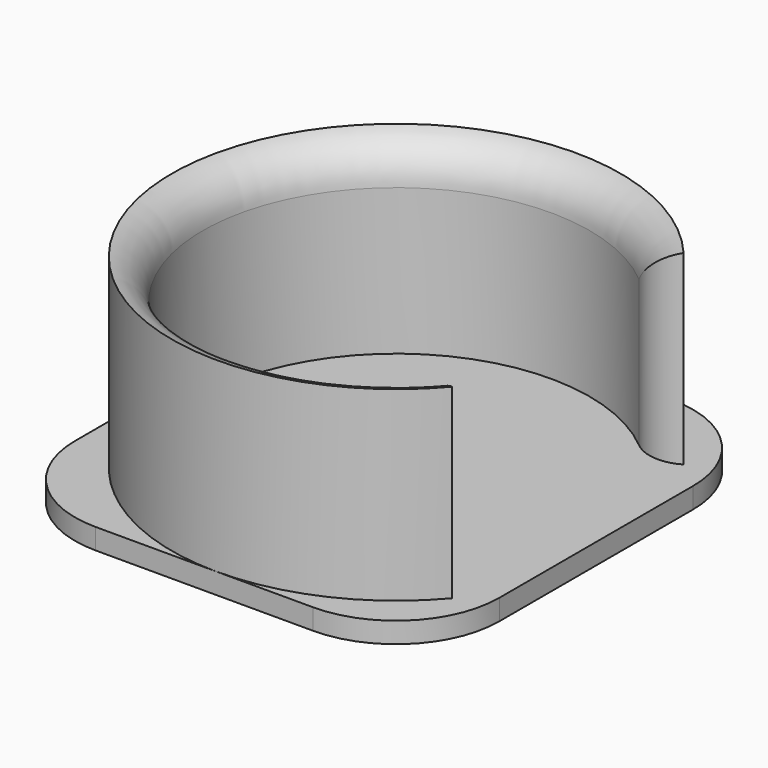
from build123d import *

# Parameters (mm, degrees)
F2_DEPTH    = 10
F3_W        = 20.5154874287
F3_H        = 21.7
F4_DEPTH    = 1
F5_R        = 5
F7_T1_DEPTH = 14.7609215151
F7_T4_ANGLE = 34.9116466648
F7_T6_ANGLE = 279.6444662417
F7_T8_ANGLE = 34.9116520269


# Not quite as in the source:
# - a fillet or chamfer that OpenCascade refuses, or shapes differently, is made with other operations: its cross-section is extruded or revolved along the edge and cut away or added


with BuildPart() as f2:
    # F0 (on Top) → F2 (new body)
    with BuildSketch(Plane.XY):
        with BuildLine():
            ThreePointArc((7.5612498967, -5.5), (-9.35, 0), (7.5612498967, 5.5))
            Line((7.5612498967, 5.5), (8.2899034976, 7))
            ThreePointArc((8.2899034976, 7), (-10.85, 0), (8.2899034976, -7))
            Line((8.2899034976, -7), (7.5612498967, -5.5))
        make_face()
    extrude(amount=F2_DEPTH)

    # F3 (on Top) → F4 (join)
    with BuildSketch(Plane.XY):
        with Locations((-0.5922562857, 0)):
            Rectangle(F3_W, F3_H)
    extrude(amount=F4_DEPTH)

    # F5
    f5_edges = [f2.edges().sort_by_distance(p)[0] for p in [
        (-10.85, -10.85, 0.5),
        (9.665487, -10.85, 0.5),
        (-10.85, 10.85, 0.5),
        (9.665487, 10.85, 0.5),
    ]]
    fillet(f5_edges, radius=F5_R)

    # F7: fillet of radius 2 on 3 edges, made by hand

    # F7_s2 → F7_t1 (cut)
    with BuildSketch(Plane.XY.offset(1)):
        with BuildLine():
            ThreePointArc((8.2899034976, 7), (7.1091806232, 6.7248281543), (5.9864319049, 7.1822790985))
            ThreePointArc((5.9864319049, 7.1822790985), (6.8258652411, 6.3898406639), (7.5612498967, 5.5))
            Line((7.5612498967, 5.5), (8.2899034976, 7))
        make_face()
        with BuildLine():
            ThreePointArc((5.9864319049, -7.1822790985), (7.1091806232, -6.7248281543), (8.2899034976, -7))
            Line((8.2899034976, -7), (7.5612498967, -5.5))
            ThreePointArc((7.5612498967, -5.5), (6.8258652411, -6.3898406639), (5.9864319049, -7.1822790985))
        make_face()
    extrude(amount=F7_T1_DEPTH, mode=Mode.SUBTRACT)

    # F7_s3 → F7_t4 (revolve, cut)
    with BuildSketch(Plane(origin=(0, 0, 0), x_dir=(0, 0, 1), z_dir=(0.091781739, 0.9957791484, 0))):
        with BuildLine():
            ThreePointArc((8, 9.35), (9.4142135624, 9.9357864376), (10, 11.35))
            Line((10, 11.35), (10, 9.35))
            Line((10, 9.35), (8, 9.35))
        make_face()
    revolve(axis=Axis((0, 0, 10), (0, 0, -1)), revolution_arc=F7_T4_ANGLE, mode=Mode.SUBTRACT)

    # F7_s5 → F7_t6 (revolve, cut)
    with BuildSketch(Plane(origin=(0, 0, 0), x_dir=(0, 0, 1), z_dir=(0.6451612191, 0.7640464655, 0))):
        with BuildLine():
            ThreePointArc((8.0635083269, 9.35), (9.2882531983, 9.7688611699), (10, 10.85))
            Line((10, 10.85), (10, 9.35))
            Line((10, 9.35), (8.0635083269, 9.35))
        make_face()
    revolve(axis=Axis((0, 0, 10), (0, 0, -1)), revolution_arc=F7_T6_ANGLE, mode=Mode.SUBTRACT)

    # F7_s7 → F7_t8 (revolve, cut)
    with BuildSketch(Plane(origin=(0, 0, 0), x_dir=(0, 0, 1), z_dir=(-0.6451612906, 0.7640464051, 0))):
        with BuildLine():
            ThreePointArc((8, 9.35), (9.4142135624, 9.9357864376), (10, 11.35))
            Line((10, 11.35), (10, 9.35))
            Line((10, 9.35), (8, 9.35))
        make_face()
    revolve(axis=Axis((0, 0, 10), (0, 0, -1)), revolution_arc=F7_T8_ANGLE, mode=Mode.SUBTRACT)


solid = f2.part
